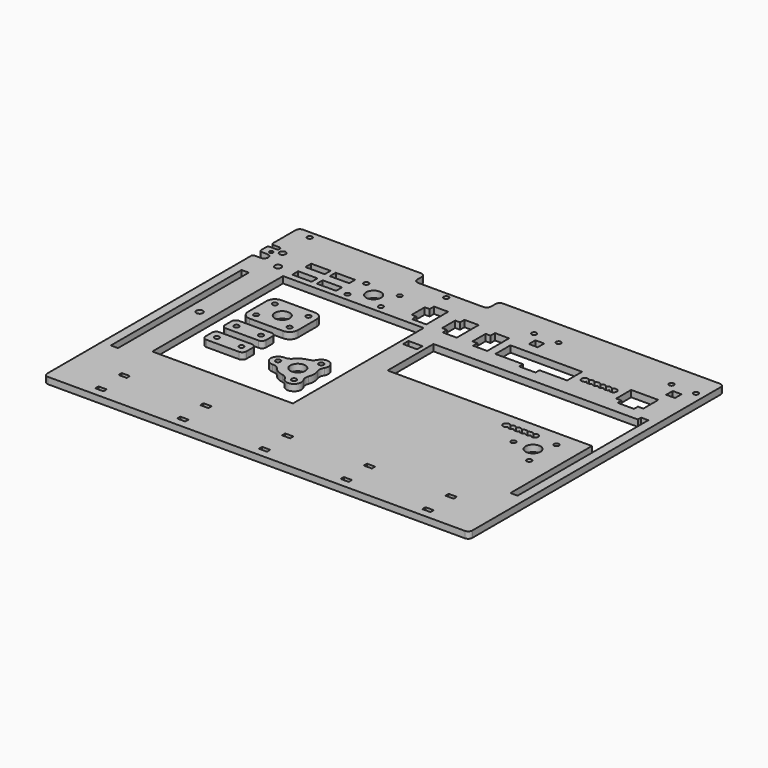
from build123d import *

# Parameters (mm, degrees)
F0_W     = 6.35
F0_H     = 3.175
F0_W_2   = 5.588
F0_H_2   = 127
F0_R     = 1.905
F0_R_2   = 5.8
F0_R_3   = 2.54
F0_W_3   = 109.22
F0_W_4   = 10.922
F0_H_3   = 5.334
F0_R_4   = 1.5
F0_R_5   = 2.375
F0_W_5   = 15
F0_H_4   = 5.75
F0_W_6   = 6.858
F0_H_5   = 6.35
F1_DEPTH = 5.08


# Not quite as in the source:
# - a feature names something its author has since deleted; it is built from what else it names


with BuildPart() as f1:
    # F0 (on Top) → F1 (new body)
    with BuildSketch(Plane.XY):
        with BuildLine():
            Line((-161.925, -111.125), (161.925, -111.125))
            ThreePointArc((161.925, -111.125), (164.1700640303, -110.1950640303), (165.1, -107.95))
            Line((165.1, -107.95), (165.1, 111.125))
            Line((165.1, 111.125), (165.1, 133.35))
            ThreePointArc((165.1, 133.35), (164.1700640303, 135.5950640303), (161.925, 136.525))
            Line((161.925, 136.525), (-6.65, 136.525))
            ThreePointArc((-6.65, 136.525), (-8.8950640303, 135.5950640303), (-9.825, 133.35))
            Line((-9.825, 133.35), (-9.825, 128.745))
            ThreePointArc((-9.825, 128.745), (-10.7549359697, 126.4999359697), (-13, 125.57))
            Line((-13, 125.57), (-63.8, 125.57))
            ThreePointArc((-63.8, 125.57), (-66.0450640303, 126.4999359697), (-66.975, 128.745))
            Line((-66.975, 128.745), (-66.975, 133.35))
            ThreePointArc((-66.975, 133.35), (-67.9049359697, 135.5950640303), (-70.15, 136.525))
            Line((-70.15, 136.525), (-161.925, 136.525))
            ThreePointArc((-161.925, 136.525), (-164.1700640303, 135.5950640303), (-165.1, 133.35))
            Line((-165.1, 133.35), (-165.1, 111.125))
            ThreePointArc((-165.1, 111.125), (-164.6350320151, 110.0024679849), (-163.5125, 109.5375))
            Line((-163.5125, 109.5375), (-158.75, 109.5375))
            ThreePointArc((-158.75, 109.5375), (-157.1625, 107.95), (-158.75, 106.3625))
            Line((-158.75, 106.3625), (-163.5125, 106.3625))
            ThreePointArc((-163.5125, 106.3625), (-164.6350320151, 105.8975320151), (-165.1, 104.775))
            Line((-165.1, 104.775), (-165.1, 99.5045))
            ThreePointArc((-165.1, 99.5045), (-164.6350320151, 98.3819679849), (-163.5125, 97.917))
            Line((-163.5125, 97.917), (-158.75, 97.917))
            ThreePointArc((-158.75, 97.917), (-155.575, 94.742), (-158.75, 91.567))
            Line((-158.75, 91.567), (-163.5125, 91.567))
            ThreePointArc((-163.5125, 91.567), (-164.6350320151, 91.1020320151), (-165.1, 89.9795))
            Line((-165.1, 89.9795), (-165.1, -107.95))
            ThreePointArc((-165.1, -107.95), (-164.1700640303, -110.1950640303), (-161.925, -111.125))
        make_face()
        with Locations((-127, -103.325)):
            Rectangle(F0_W, F0_H, mode=Mode.SUBTRACT)
        with Locations((-127, -80.825)):
            Rectangle(F0_W, F0_H, mode=Mode.SUBTRACT)
        with Locations((-63.5, -103.325)):
            Rectangle(F0_W, F0_H, mode=Mode.SUBTRACT)
        with Locations((-63.5, -80.825)):
            Rectangle(F0_W, F0_H, mode=Mode.SUBTRACT)
        with Locations((-155.194, 8.4074)):
            Rectangle(F0_W_2, F0_H_2, mode=Mode.SUBTRACT)
        with Locations((0, -103.325)):
            Rectangle(F0_W, F0_H, mode=Mode.SUBTRACT)
        with Locations((0, -80.825)):
            Rectangle(F0_W, F0_H, mode=Mode.SUBTRACT)
        with Locations((63.5, -103.325)):
            Rectangle(F0_W, F0_H, mode=Mode.SUBTRACT)
        with Locations((63.5, -80.825)):
            Rectangle(F0_W, F0_H, mode=Mode.SUBTRACT)
        with Locations((127, -103.325)):
            Rectangle(F0_W, F0_H, mode=Mode.SUBTRACT)
        with Locations((127, -80.825)):
            Rectangle(F0_W, F0_H, mode=Mode.SUBTRACT)
        Polygon((-6.35, 68.707), (152.4, 68.707), (152.4, 71.9074), (157.988, 71.9074), (157.988, -55.0926), (152.4, -55.0926), (152.4, 24.1046), (-6.35, 24.1046), align=None, mode=Mode.SUBTRACT)
        with Locations((111.76, -1.2954)):
            Circle(F0_R, mode=Mode.SUBTRACT)
        with Locations((134.62, -14.4936271537)):
            Circle(F0_R, mode=Mode.SUBTRACT)
        with Locations((127, -1.2954)):
            Circle(F0_R_2, mode=Mode.SUBTRACT)
        with Locations((134.62, 11.9028271537)):
            Circle(F0_R, mode=Mode.SUBTRACT)
        with Locations((-143.51, 13.0175)):
            Circle(F0_R_3, mode=Mode.SUBTRACT)
        with Locations((-78.74, 17.907)):
            Rectangle(F0_W_3, F0_H_2, mode=Mode.SUBTRACT)
        with Locations((-15.24, 59.69)):
            Rectangle(F0_W_4, F0_H_3, mode=Mode.SUBTRACT)
        with Locations((-143.51, 89.2175)):
            Circle(F0_R_3, mode=Mode.SUBTRACT)
        with Locations((-158.75, 101.6)):
            Circle(F0_R_4, mode=Mode.SUBTRACT)
        with Locations((-152.4, 104.775)):
            Circle(F0_R_5, mode=Mode.SUBTRACT)
        with Locations((-122.675, 89.2)):
            Rectangle(F0_W_5, F0_H_4, mode=Mode.SUBTRACT)
        with Locations((-103.625, 89.2)):
            Rectangle(F0_W_5, F0_H_4, mode=Mode.SUBTRACT)
        with Locations((-87.9340387031, 87.1604740729)):
            Circle(F0_R, mode=Mode.SUBTRACT)
        with Locations((-122.675, 101.9)):
            Rectangle(F0_W_5, F0_H_4, mode=Mode.SUBTRACT)
        with Locations((-103.625, 101.9)):
            Rectangle(F0_W_5, F0_H_4, mode=Mode.SUBTRACT)
        with Locations((-87.9340387031, 105.3715259271)):
            Circle(F0_R, mode=Mode.SUBTRACT)
        with Locations((-152.4, 131.125)):
            Circle(F0_R, mode=Mode.SUBTRACT)
        with Locations((-61.9259612969, 87.1604740729)):
            Circle(F0_R, mode=Mode.SUBTRACT)
        with Locations((-74.93, 96.266)):
            Circle(F0_R_2, mode=Mode.SUBTRACT)
        with Locations((-61.9259612969, 105.3715259271)):
            Circle(F0_R, mode=Mode.SUBTRACT)
        Polygon((-36.8271034363, 90.34), (-40.6371034363, 90.34), (-40.6371034363, 103.04), (-36.8271034363, 103.04), (-36.8271034363, 107.315), (-25.8271034363, 107.315), (-25.8271034363, 86.065), (-36.8271034363, 86.065), align=None, mode=Mode.SUBTRACT)
        Polygon((-11.5120017181, 88.265), (-15.3220017181, 88.265), (-15.3220017181, 100.965), (-11.5120017181, 100.965), (-11.5120017181, 105.24), (-0.5120017181, 105.24), (-0.5120017181, 83.99), (-11.5120017181, 83.99), align=None, mode=Mode.SUBTRACT)
        with Locations((-38.4, 121.125)):
            Circle(F0_R, mode=Mode.SUBTRACT)
        with BuildLine():
            ThreePointArc((110.363, 14.2471722124), (112.5855, 15.5575), (114.808, 14.2471722124))
            ThreePointArc((114.808, 14.2471722124), (119.5705, 13.0175), (114.808, 11.7878277876))
            ThreePointArc((114.808, 11.7878277876), (112.5855, 10.4775), (110.363, 11.7878277876))
            ThreePointArc((110.363, 11.7878277876), (108.1405, 10.4775), (105.918, 11.7878277876))
            ThreePointArc((105.918, 11.7878277876), (103.6955, 10.4775), (101.473, 11.7878277876))
            ThreePointArc((101.473, 11.7878277876), (99.2505, 10.4775), (97.028, 11.7878277876))
            ThreePointArc((97.028, 11.7878277876), (92.2655, 13.0175), (97.028, 14.2471722124))
            ThreePointArc((97.028, 14.2471722124), (99.2505, 15.5575), (101.473, 14.2471722124))
            ThreePointArc((101.473, 14.2471722124), (103.6955, 15.5575), (105.918, 14.2471722124))
            ThreePointArc((105.918, 14.2471722124), (108.1405, 15.5575), (110.363, 14.2471722124))
        make_face(mode=Mode.SUBTRACT)
        Polygon((13.8031, 98.89), (13.8031, 103.165), (24.8031, 103.165), (24.8031, 81.915), (13.8031, 81.915), (13.8031, 86.19), (9.9931, 86.19), (9.9931, 98.89), align=None, mode=Mode.SUBTRACT)
        Polygon((31.1531, 96.52), (86.868, 96.52), (86.868, 81.915), (65.36055, 81.915), (65.36055, 78.105), (52.66055, 78.105), (52.66055, 81.915), (31.1531, 81.915), align=None, mode=Mode.SUBTRACT)
        with Locations((32.766, 117.475)):
            Circle(F0_R, mode=Mode.SUBTRACT)
        with Locations((42.291, 107.95)):
            Rectangle(F0_W_6, F0_H_5, mode=Mode.SUBTRACT)
        with Locations((51.816, 117.475)):
            Circle(F0_R, mode=Mode.SUBTRACT)
        with BuildLine():
            ThreePointArc((97.028, 87.9878277876), (92.2655, 89.2175), (97.028, 90.4471722124))
            ThreePointArc((97.028, 90.4471722124), (99.2505, 91.7575), (101.473, 90.4471722124))
            ThreePointArc((101.473, 90.4471722124), (103.6955, 91.7575), (105.918, 90.4471722124))
            ThreePointArc((105.918, 90.4471722124), (108.1405, 91.7575), (110.363, 90.4471722124))
            ThreePointArc((110.363, 90.4471722124), (112.5855, 91.7575), (114.808, 90.4471722124))
            ThreePointArc((114.808, 90.4471722124), (119.5705, 89.2175), (114.808, 87.9878277876))
            ThreePointArc((114.808, 87.9878277876), (112.5855, 86.6775), (110.363, 87.9878277876))
            ThreePointArc((110.363, 87.9878277876), (108.1405, 86.6775), (105.918, 87.9878277876))
            ThreePointArc((105.918, 87.9878277876), (103.6955, 86.6775), (101.473, 87.9878277876))
            ThreePointArc((101.473, 87.9878277876), (99.2505, 86.6775), (97.028, 87.9878277876))
        make_face(mode=Mode.SUBTRACT)
        Polygon((124.968, 96.52), (146.05, 96.52), (146.05, 81.915), (141.859, 81.915), (141.859, 78.105), (129.159, 78.105), (129.159, 81.915), (124.968, 81.915), align=None, mode=Mode.SUBTRACT)
        with Locations((139.446, 117.475)):
            Circle(F0_R, mode=Mode.SUBTRACT)
        with Locations((148.971, 107.95)):
            Rectangle(F0_W_6, F0_H_5, mode=Mode.SUBTRACT)
        with Locations((158.496, 117.475)):
            Circle(F0_R, mode=Mode.SUBTRACT)
    extrude(amount=F1_DEPTH)


with BuildPart() as f1b:
    # F0 (on Top) → F1, piece 2 (new body)
    with BuildSketch(Plane.XY):
        with BuildLine():
            ThreePointArc((-81.9419225938, 49.657), (-83.8017945333, 54.1471280605), (-88.2919225938, 56.007))
            Line((-88.2919225938, 56.007), (-114.3, 56.007))
            ThreePointArc((-114.3, 56.007), (-118.7901280605, 54.1471280605), (-120.65, 49.657))
            Line((-120.65, 49.657), (-120.65, 31.4459481459))
            ThreePointArc((-120.65, 31.4459481459), (-118.7901280605, 26.9558200853), (-114.3, 25.0959481459))
            Line((-114.3, 25.0959481459), (-88.2919225938, 25.0959481459))
            ThreePointArc((-88.2919225938, 25.0959481459), (-83.8017945333, 26.9558200853), (-81.9419225938, 31.4459481459))
            Line((-81.9419225938, 31.4459481459), (-81.9419225938, 49.657))
        make_face()
        with Locations((-114.3, 31.4459481459)):
            Circle(F0_R, mode=Mode.SUBTRACT)
        with Locations((-88.2919225938, 31.4459481459)):
            Circle(F0_R, mode=Mode.SUBTRACT)
        with Locations((-101.2959612969, 40.5514740729)):
            Circle(F0_R_2, mode=Mode.SUBTRACT)
        with Locations((-114.3, 49.657)):
            Circle(F0_R, mode=Mode.SUBTRACT)
        with Locations((-88.2919225938, 49.657)):
            Circle(F0_R, mode=Mode.SUBTRACT)
    extrude(amount=F1_DEPTH)


with BuildPart() as f1c:
    # F0 (on Top) → F1, piece 3 (new body)
    with BuildSketch(Plane.XY):
        with BuildLine():
            Line((-92.075, 18.7459481459), (-117.475, 18.7459481459))
            ThreePointArc((-117.475, 18.7459481459), (-119.7200640303, 17.8160121761), (-120.65, 15.5709481459))
            Line((-120.65, 15.5709481459), (-120.65, 9.2209481459))
            ThreePointArc((-120.65, 9.2209481459), (-119.7200640303, 6.9758841156), (-117.475, 6.0459481459))
            Line((-117.475, 6.0459481459), (-92.075, 6.0459481459))
            ThreePointArc((-92.075, 6.0459481459), (-89.8299359697, 6.9758841156), (-88.9, 9.2209481459))
            Line((-88.9, 9.2209481459), (-88.9, 15.5709481459))
            ThreePointArc((-88.9, 15.5709481459), (-89.8299359697, 17.8160121761), (-92.075, 18.7459481459))
        make_face()
        with Locations((-114.3, 12.3959481459)):
            Circle(F0_R, mode=Mode.SUBTRACT)
        with Locations((-95.25, 12.3959481459)):
            Circle(F0_R, mode=Mode.SUBTRACT)
    extrude(amount=F1_DEPTH)


with BuildPart() as f1d:
    # F0 (on Top) → F1, piece 4 (new body)
    with BuildSketch(Plane.XY):
        with BuildLine():
            Line((-120.65, -3.4790518541), (-120.65, -9.8290518541))
            ThreePointArc((-120.65, -9.8290518541), (-119.7200640303, -12.0741158844), (-117.475, -13.0040518541))
            Line((-117.475, -13.0040518541), (-92.075, -13.0040518541))
            ThreePointArc((-92.075, -13.0040518541), (-89.8299359697, -12.0741158844), (-88.9, -9.8290518541))
            Line((-88.9, -9.8290518541), (-88.9, -3.4790518541))
            ThreePointArc((-88.9, -3.4790518541), (-89.8299359697, -1.2339878239), (-92.075, -0.3040518541))
            Line((-92.075, -0.3040518541), (-117.475, -0.3040518541))
            ThreePointArc((-117.475, -0.3040518541), (-119.7200640303, -1.2339878239), (-120.65, -3.4790518541))
        make_face()
        with Locations((-114.3, -6.6540518541)):
            Circle(F0_R, mode=Mode.SUBTRACT)
        with Locations((-95.25, -6.6540518541)):
            Circle(F0_R, mode=Mode.SUBTRACT)
    extrude(amount=F1_DEPTH)


with BuildPart() as f1e:
    # F0 (on Top) → F1, piece 5 (new body)
    with BuildSketch(Plane.XY):
        with BuildLine():
            ThreePointArc((-60.6336805556, 0.5437111887), (-62.9466515429, -1.2295102662), (-65.8081414474, -1.782705208))
            ThreePointArc((-65.8081414474, -1.782705208), (-71.755, -7.493), (-65.8081414474, -13.203294792))
            ThreePointArc((-65.8081414474, -13.203294792), (-62.9466515429, -13.7564897338), (-60.6336805556, -15.5297111887))
            ThreePointArc((-60.6336805556, -15.5297111887), (-57.15, -18.4915226281), (-52.8431557746, -20.0275727682))
            ThreePointArc((-52.8431557746, -20.0275727682), (-50.1510154543, -21.144053674), (-48.2411896293, -23.345579153))
            ThreePointArc((-48.2411896293, -23.345579153), (-40.3225, -25.6405623363), (-38.3506689233, -17.635284361))
            ThreePointArc((-38.3506689233, -17.635284361), (-39.3023330027, -14.8805639402), (-38.9231636699, -11.9908615794))
            ThreePointArc((-38.9231636699, -11.9908615794), (-38.1, -7.493), (-38.9231636699, -2.9951384206))
            ThreePointArc((-38.9231636699, -2.9951384206), (-39.3023330027, -0.1054360598), (-38.3506689233, 2.649284361))
            ThreePointArc((-38.3506689233, 2.649284361), (-40.3225, 10.6545623363), (-48.2411896293, 8.359579153))
            ThreePointArc((-48.2411896293, 8.359579153), (-50.1510154543, 6.158053674), (-52.8431557746, 5.0415727682))
            ThreePointArc((-52.8431557746, 5.0415727682), (-57.15, 3.5055226281), (-60.6336805556, 0.5437111887))
        make_face()
        with Locations((-43.18, -20.6912271537)):
            Circle(F0_R, mode=Mode.SUBTRACT)
        with Locations((-66.04, -7.493)):
            Circle(F0_R, mode=Mode.SUBTRACT)
        with Locations((-50.8, -7.493)):
            Circle(F0_R_2, mode=Mode.SUBTRACT)
        with Locations((-43.18, 5.7052271537)):
            Circle(F0_R, mode=Mode.SUBTRACT)
    extrude(amount=F1_DEPTH)


solid = Compound([f1.part, f1b.part, f1c.part, f1d.part, f1e.part])
